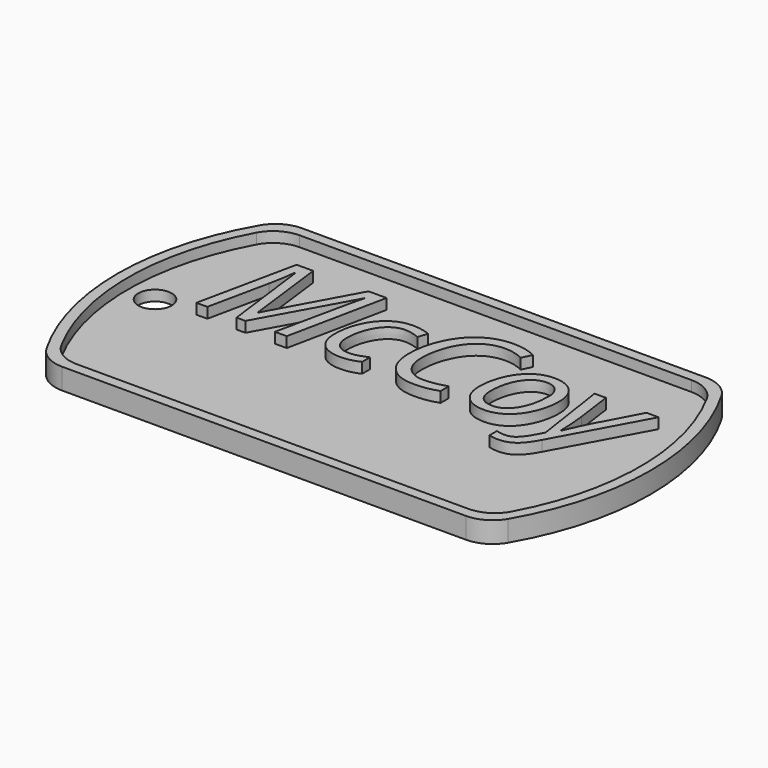
from build123d import *

# Parameters (mm, degrees)
F1_DEPTH     = 1
F3_DEPTH     = 1
F4_R         = 1.5875
F5_DEPTH     = 1
F6_TEXT_SIZE = 13.2295096086
F7_DEPTH     = 1


# Not quite as in the source:
# - Text() gives the source's letters only with a copy of the font that has no kerning and outlines rounded to 1/6400 em; it was checked with that copy


with BuildPart() as f1:
    # F0 (on Top) → F1 (new body)
    with BuildSketch(Plane.XY):
        with BuildLine():
            ThreePointArc((-19.2474145991, 14.2875), (-20.8349145991, 13.862130657), (-21.9970452561, 12.7))
            ThreePointArc((-21.9970452561, 12.7), (-25.4, 0), (-21.9970452561, -12.7))
            ThreePointArc((-21.9970452561, -12.7), (-20.8349145991, -13.862130657), (-19.2474145991, -14.2875))
            Line((-19.2474145991, -14.2875), (19.2474145991, -14.2875))
            ThreePointArc((19.2474145991, -14.2875), (20.8349145991, -13.862130657), (21.9970452561, -12.7))
            ThreePointArc((21.9970452561, -12.7), (25.4, 0), (21.9970452561, 12.7))
            ThreePointArc((21.9970452561, 12.7), (20.8349145991, 13.862130657), (19.2474145991, 14.2875))
            Line((19.2474145991, 14.2875), (-19.2474145991, 14.2875))
        make_face()
    extrude(amount=F1_DEPTH)

    # F2 (on face) → F3 (join)
    with BuildSketch(Plane.XY.offset(1)):
        with BuildLine():
            Line((19.2474145991, 14.2875), (-19.2474145991, 14.2875))
            ThreePointArc((-19.2474145991, 14.2875), (-20.8349145991, 13.862130657), (-21.9970452561, 12.7))
            ThreePointArc((-21.9970452561, 12.7), (-25.4, 0), (-21.9970452561, -12.7))
            ThreePointArc((-21.9970452561, -12.7), (-20.8349145991, -13.862130657), (-19.2474145991, -14.2875))
            Line((-19.2474145991, -14.2875), (19.2474145991, -14.2875))
            ThreePointArc((19.2474145991, -14.2875), (20.8349145991, -13.862130657), (21.9970452561, -12.7))
            ThreePointArc((21.9970452561, -12.7), (25.4, 0), (21.9970452561, 12.7))
            ThreePointArc((21.9970452561, 12.7), (20.8349145991, 13.862130657), (19.2474145991, 14.2875))
        make_face()
        with BuildLine():
            ThreePointArc((-21.4526124879, 11.6252061249), (-20.2856017842, 12.8404540819), (-18.6611352482, 13.2875))
            Line((-18.6611352482, 13.2875), (18.6611352482, 13.2875))
            ThreePointArc((18.6611352482, 13.2875), (20.2856017842, 12.8404540819), (21.4526124879, 11.6252061249))
            ThreePointArc((21.4526124879, 11.6252061249), (24.4, 0), (21.4526124879, -11.6252061249))
            ThreePointArc((21.4526124879, -11.6252061249), (20.2856017842, -12.8404540819), (18.6611352482, -13.2875))
            Line((18.6611352482, -13.2875), (-18.6611352482, -13.2875))
            ThreePointArc((-18.6611352482, -13.2875), (-20.2856017842, -12.8404540819), (-21.4526124879, -11.6252061249))
            ThreePointArc((-21.4526124879, -11.6252061249), (-24.4, 0), (-21.4526124879, 11.6252061249))
        make_face(mode=Mode.SUBTRACT)
    extrude(amount=F3_DEPTH)

    # F4 (on face) → F5 (cut)
    with BuildSketch(Plane.XY.offset(1)):
        with Locations((-21.821282804, 0)):
            Circle(F4_R)
    extrude(amount=-F5_DEPTH, mode=Mode.SUBTRACT)

    # F6 (on face) → F7 (join)
    with BuildSketch(Plane.XY.offset(1)):
        with Locations((-18.4208950959, 0)):
            Text('McCoy', F6_TEXT_SIZE, font='Open Sans', font_style=FontStyle.ITALIC, text_align=(TextAlign.LEFT, TextAlign.BOTTOM))
    extrude(amount=F7_DEPTH)


solid = f1.part
